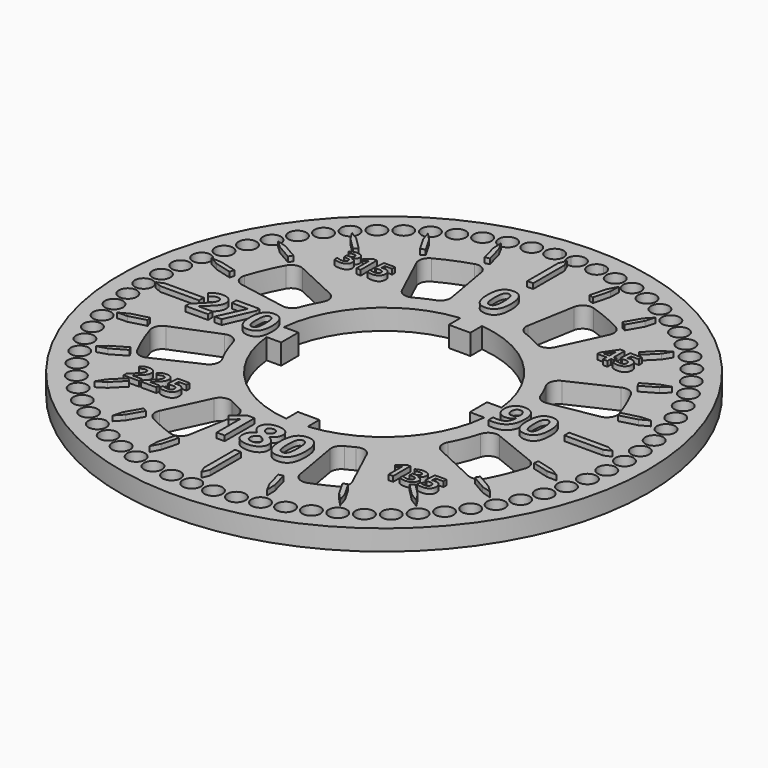
from build123d import *

# Parameters (mm, degrees)
F0_R           = 51.5
F0_R_2         = 1.75
F1_DEPTH       = 4
F3_TEXT_SIZE   = 9.3811322909
F3_TEXT_SIZE_2 = 9.1976195108
F3_TEXT_SIZE_3 = 10.2249465676
F3_TEXT_SIZE_4 = 8.8090639717
F4_DEPTH       = 1
F5_TEXT_SIZE   = 5.8529381123
F5_TEXT_SIZE_2 = 5.8596281128
F5_TEXT_SIZE_3 = 5.9887766838
F5_TEXT_SIZE_4 = 5.5610072903
F6_DEPTH       = 1
F8_DEPTH       = 4.001
F9_R           = 2


# Not quite as in the source:
# - Text() gives the source's letters only with a copy of the font that has no kerning and outlines rounded to 1/6400 em; it was checked with that copy


with BuildPart() as f1:
    # F0 (on Top) → F1 (new body)
    with BuildSketch(Plane.XY):
        Circle(F0_R)
        with Locations((-33.1633080376, -33.1633080376)):
            Circle(F0_R_2, mode=Mode.SUBTRACT)
        with Locations((-30.1467388943, -35.9274843823)):
            Circle(F0_R_2, mode=Mode.SUBTRACT)
        with Locations((-26.9007348649, -38.4182308772)):
            Circle(F0_R_2, mode=Mode.SUBTRACT)
        with Locations((-35.9274843823, -30.1467388943)):
            Circle(F0_R_2, mode=Mode.SUBTRACT)
        with Locations((-38.4182308772, -26.9007348649)):
            Circle(F0_R_2, mode=Mode.SUBTRACT)
        with Locations((-19.8207964756, -42.505835212)):
            Circle(F0_R_2, mode=Mode.SUBTRACT)
        with Locations((-23.45, -40.6165914375)):
            Circle(F0_R_2, mode=Mode.SUBTRACT)
        with Locations((-16.040744722, -44.0715839149)):
            Circle(F0_R_2, mode=Mode.SUBTRACT)
        with Locations((-12.1386132153, -45.301921253)):
            Circle(F0_R_2, mode=Mode.SUBTRACT)
        with Locations((-8.1440995326, -46.1874836163)):
            Circle(F0_R_2, mode=Mode.SUBTRACT)
        with Locations((-4.0876043349, -46.7215313405)):
            Circle(F0_R_2, mode=Mode.SUBTRACT)
        with Locations((0, -46.9)):
            Circle(F0_R_2, mode=Mode.SUBTRACT)
        with Locations((-40.6165914375, -23.45)):
            Circle(F0_R_2, mode=Mode.SUBTRACT)
        with Locations((-42.505835212, -19.8207964756)):
            Circle(F0_R_2, mode=Mode.SUBTRACT)
        with Locations((-44.0715839149, -16.040744722)):
            Circle(F0_R_2, mode=Mode.SUBTRACT)
        with Locations((-45.301921253, -12.1386132153)):
            Circle(F0_R_2, mode=Mode.SUBTRACT)
        with Locations((-46.1874836163, -8.1440995326)):
            Circle(F0_R_2, mode=Mode.SUBTRACT)
        with Locations((-46.7215313405, -4.0876043349)):
            Circle(F0_R_2, mode=Mode.SUBTRACT)
        with Locations((-46.9, 0)):
            Circle(F0_R_2, mode=Mode.SUBTRACT)
        with Locations((4.0876043349, -46.7215313405)):
            Circle(F0_R_2, mode=Mode.SUBTRACT)
        with Locations((8.1440995326, -46.1874836163)):
            Circle(F0_R_2, mode=Mode.SUBTRACT)
        with Locations((12.1386132153, -45.301921253)):
            Circle(F0_R_2, mode=Mode.SUBTRACT)
        with Locations((16.040744722, -44.0715839149)):
            Circle(F0_R_2, mode=Mode.SUBTRACT)
        with Locations((19.8207964756, -42.505835212)):
            Circle(F0_R_2, mode=Mode.SUBTRACT)
        with Locations((23.45, -40.6165914375)):
            Circle(F0_R_2, mode=Mode.SUBTRACT)
        with Locations((26.9007348649, -38.4182308772)):
            Circle(F0_R_2, mode=Mode.SUBTRACT)
        with Locations((30.1467388943, -35.9274843823)):
            Circle(F0_R_2, mode=Mode.SUBTRACT)
        with Locations((33.1633080376, -33.1633080376)):
            Circle(F0_R_2, mode=Mode.SUBTRACT)
        with Locations((35.9274843823, -30.1467388943)):
            Circle(F0_R_2, mode=Mode.SUBTRACT)
        with Locations((38.4182308772, -26.9007348649)):
            Circle(F0_R_2, mode=Mode.SUBTRACT)
        with Locations((40.6165914375, -23.45)):
            Circle(F0_R_2, mode=Mode.SUBTRACT)
        with Locations((42.505835212, -19.8207964756)):
            Circle(F0_R_2, mode=Mode.SUBTRACT)
        with Locations((44.0715839149, -16.040744722)):
            Circle(F0_R_2, mode=Mode.SUBTRACT)
        with Locations((45.301921253, -12.1386132153)):
            Circle(F0_R_2, mode=Mode.SUBTRACT)
        with Locations((46.1874836163, -8.1440995326)):
            Circle(F0_R_2, mode=Mode.SUBTRACT)
        with Locations((46.7215313405, -4.0876043349)):
            Circle(F0_R_2, mode=Mode.SUBTRACT)
        with Locations((46.9, 0)):
            Circle(F0_R_2, mode=Mode.SUBTRACT)
        with Locations((-46.7215313405, 4.0876043349)):
            Circle(F0_R_2, mode=Mode.SUBTRACT)
        with Locations((-46.1874836163, 8.1440995326)):
            Circle(F0_R_2, mode=Mode.SUBTRACT)
        with Locations((-45.301921253, 12.1386132153)):
            Circle(F0_R_2, mode=Mode.SUBTRACT)
        with Locations((-44.0715839149, 16.040744722)):
            Circle(F0_R_2, mode=Mode.SUBTRACT)
        with Locations((-42.505835212, 19.8207964756)):
            Circle(F0_R_2, mode=Mode.SUBTRACT)
        with Locations((-40.6165914375, 23.45)):
            Circle(F0_R_2, mode=Mode.SUBTRACT)
        with BuildLine():
            Line((1.6706053866, 42.8881468691), (1.6706053866, 42.2931905308))
            ThreePointArc((1.6706053866, 42.2931905308), (30.5140559381, 29.3325293461), (42.3261726079, 0))
            ThreePointArc((42.3261726079, 0), (-29.3552011859, -30.4922457514), (-1.6077337049, 42.2956271967))
            Line((-1.6077337049, 42.2956271967), (-1.6077337049, 42.8625403735))
            ThreePointArc((-1.6077337049, 42.8625403735), (-2.9504268896, 43.7092525844), (-3.8994754635, 44.9816728613))
            ThreePointArc((-3.8994754635, 44.9816728613), (-5.8359387226, 46.6451974126), (-4.0518300087, 48.4711656445))
            ThreePointArc((-4.0518300087, 48.4711656445), (0, 51.2457896753), (4.0518300087, 48.4711656445))
            ThreePointArc((4.0518300087, 48.4711656445), (5.3123277586, 47.9715523545), (5.8376043349, 46.7215313405))
            ThreePointArc((5.8376043349, 46.7215313405), (5.2566369424, 45.4192783841), (3.8994754635, 44.9816728613))
            ThreePointArc((3.8994754635, 44.9816728613), (2.9752584659, 43.7323944434), (1.6706053866, 42.8881468691))
        make_face(mode=Mode.SUBTRACT)
        with Locations((-38.4182308772, 26.9007348649)):
            Circle(F0_R_2, mode=Mode.SUBTRACT)
        with Locations((-35.9274843823, 30.1467388943)):
            Circle(F0_R_2, mode=Mode.SUBTRACT)
        with Locations((-33.1633080376, 33.1633080376)):
            Circle(F0_R_2, mode=Mode.SUBTRACT)
        with Locations((-30.1467388943, 35.9274843823)):
            Circle(F0_R_2, mode=Mode.SUBTRACT)
        with Locations((-26.9007348649, 38.4182308772)):
            Circle(F0_R_2, mode=Mode.SUBTRACT)
        with Locations((-23.45, 40.6165914375)):
            Circle(F0_R_2, mode=Mode.SUBTRACT)
        with Locations((-19.8207964756, 42.505835212)):
            Circle(F0_R_2, mode=Mode.SUBTRACT)
        with Locations((-16.040744722, 44.0715839149)):
            Circle(F0_R_2, mode=Mode.SUBTRACT)
        with Locations((-12.1386132153, 45.301921253)):
            Circle(F0_R_2, mode=Mode.SUBTRACT)
        with Locations((-8.1440995326, 46.1874836163)):
            Circle(F0_R_2, mode=Mode.SUBTRACT)
        with Locations((46.7215313405, 4.0876043349)):
            Circle(F0_R_2, mode=Mode.SUBTRACT)
        with Locations((46.1874836163, 8.1440995326)):
            Circle(F0_R_2, mode=Mode.SUBTRACT)
        with Locations((45.301921253, 12.1386132153)):
            Circle(F0_R_2, mode=Mode.SUBTRACT)
        with Locations((44.0715839149, 16.040744722)):
            Circle(F0_R_2, mode=Mode.SUBTRACT)
        with Locations((42.505835212, 19.8207964756)):
            Circle(F0_R_2, mode=Mode.SUBTRACT)
        with Locations((40.6165914375, 23.45)):
            Circle(F0_R_2, mode=Mode.SUBTRACT)
        with Locations((8.1440995326, 46.1874836163)):
            Circle(F0_R_2, mode=Mode.SUBTRACT)
        with Locations((12.1386132153, 45.301921253)):
            Circle(F0_R_2, mode=Mode.SUBTRACT)
        with Locations((16.040744722, 44.0715839149)):
            Circle(F0_R_2, mode=Mode.SUBTRACT)
        with Locations((23.45, 40.6165914375)):
            Circle(F0_R_2, mode=Mode.SUBTRACT)
        with Locations((19.8207964756, 42.505835212)):
            Circle(F0_R_2, mode=Mode.SUBTRACT)
        with Locations((38.4182308772, 26.9007348649)):
            Circle(F0_R_2, mode=Mode.SUBTRACT)
        with Locations((35.9274843823, 30.1467388943)):
            Circle(F0_R_2, mode=Mode.SUBTRACT)
        with Locations((26.9007348649, 38.4182308772)):
            Circle(F0_R_2, mode=Mode.SUBTRACT)
        with Locations((30.1467388943, 35.9274843823)):
            Circle(F0_R_2, mode=Mode.SUBTRACT)
        with Locations((33.1633080376, 33.1633080376)):
            Circle(F0_R_2, mode=Mode.SUBTRACT)
        with BuildLine():
            Line((1.6706053866, 46.3788688819), (1.6706053866, 42.8881468691))
            ThreePointArc((1.6706053866, 42.8881468691), (2.9752584659, 43.7323944434), (3.8994754635, 44.9816728613))
            ThreePointArc((3.8994754635, 44.9816728613), (2.3392699471, 46.7978652684), (4.0518300087, 48.4711656445))
            ThreePointArc((4.0518300087, 48.4711656445), (0, 51.2457896753), (-4.0518300087, 48.4711656445))
            ThreePointArc((-4.0518300087, 48.4711656445), (-2.8375833209, 47.9462547642), (-2.3376043349, 46.7215313405))
            ThreePointArc((-2.3376043349, 46.7215313405), (-2.7853513785, 45.5524987329), (-3.8994754635, 44.9816728613))
            ThreePointArc((-3.8994754635, 44.9816728613), (-2.9504268896, 43.7092525844), (-1.6077337049, 42.8625403735))
            Line((-1.6077337049, 42.8625403735), (-1.6077337049, 46.2088470978))
            ThreePointArc((-1.6077337049, 46.2088470978), (-1.75, 46.9), (-1.6077337049, 47.5911529022))
            Line((-1.6077337049, 47.5911529022), (-1.6077337049, 48.9033423511))
            Line((-1.6077337049, 48.9033423511), (1.6706053866, 48.9033423511))
            Line((1.6706053866, 48.9033423511), (1.6706053866, 47.4211311181))
            ThreePointArc((1.6706053866, 47.4211311181), (1.730037489, 47.1635721661), (1.75, 46.9))
            ThreePointArc((1.75, 46.9), (1.730037489, 46.6364278339), (1.6706053866, 46.3788688819))
        make_face()
        with BuildLine():
            ThreePointArc((-1.6077337049, 42.8625403735), (0.0339431178, 42.5543428844), (1.6706053866, 42.8881468691))
            Line((1.6706053866, 42.8881468691), (1.6706053866, 46.3788688819))
            ThreePointArc((1.6706053866, 46.3788688819), (0.0906369895, 45.1523487373), (-1.6077337049, 46.2088470978))
            Line((-1.6077337049, 46.2088470978), (-1.6077337049, 42.8625403735))
        make_face()
        with BuildLine():
            ThreePointArc((-1.6077337049, 47.5911529022), (0.0906369895, 48.6476512627), (1.6706053866, 47.4211311181))
            Line((1.6706053866, 47.4211311181), (1.6706053866, 48.9033423511))
            Line((1.6706053866, 48.9033423511), (-1.6077337049, 48.9033423511))
            Line((-1.6077337049, 48.9033423511), (-1.6077337049, 47.5911529022))
        make_face()
        with BuildLine():
            ThreePointArc((-1.6077337049, 24.5811957581), (0.0315056688, 24.633696433), (1.6706053866, 24.5770028727))
            Line((1.6706053866, 24.5770028727), (1.6706053866, 27.6260756154))
            ThreePointArc((1.6706053866, 27.6260756154), (0.0314911204, 27.6765240696), (-1.6077337049, 27.629805801))
            Line((-1.6077337049, 27.629805801), (-1.6077337049, 24.5811957581))
        make_face()
        with BuildLine():
            ThreePointArc((-1.6077337049, 24.5811957581), (-16.840658184, -17.9781040294), (24.6337165804, 0))
            ThreePointArc((24.6337165804, 0), (17.999627943, 16.8176510392), (1.6706053866, 24.5770028727))
            ThreePointArc((1.6706053866, 24.5770028727), (0.0315056688, 24.633696433), (-1.6077337049, 24.5811957581))
        make_face()
        with BuildLine():
            ThreePointArc((21.2464702951, 2.1), (21.3241018662, 1.0512752256), (21.35, 0))
            ThreePointArc((21.35, 0), (21.3241018662, -1.0512752256), (21.2464702951, -2.1))
            ThreePointArc((21.2464702951, -2.1), (15.0967297783, -15.0967297783), (2.1, -21.2464702951))
            ThreePointArc((2.1, -21.2464702951), (0, -21.35), (-2.1, -21.2464702951))
            ThreePointArc((-2.1, -21.2464702951), (-15.0967297783, -15.0967297783), (-21.2464702951, -2.1))
            ThreePointArc((-21.2464702951, -2.1), (-21.35, 0), (-21.2464702951, 2.1))
            ThreePointArc((-21.2464702951, 2.1), (-15.0967297783, 15.0967297783), (-2.1, 21.2464702951))
            ThreePointArc((-2.1, 21.2464702951), (0, 21.35), (2.1, 21.2464702951))
            ThreePointArc((2.1, 21.2464702951), (15.0967297783, 15.0967297783), (21.2464702951, 2.1))
        make_face(mode=Mode.SUBTRACT)
        with BuildLine():
            Line((-18.4065936816, 2.1), (-21.2464702951, 2.1))
            ThreePointArc((-21.2464702951, 2.1), (-21.35, 0), (-21.2464702951, -2.1))
            Line((-21.2464702951, -2.1), (-18.4065936816, -2.1))
            Line((-18.4065936816, -2.1), (-18.4065936816, 2.1))
        make_face()
        with BuildLine():
            Line((2.1, 18.4065936816), (2.1, 21.2464702951))
            ThreePointArc((2.1, 21.2464702951), (0, 21.35), (-2.1, 21.2464702951))
            Line((-2.1, 21.2464702951), (-2.1, 18.4065936816))
            Line((-2.1, 18.4065936816), (2.1, 18.4065936816))
        make_face()
        with BuildLine():
            ThreePointArc((21.2464702951, -2.1), (21.3241018662, -1.0512752256), (21.35, 0))
            ThreePointArc((21.35, 0), (21.3241018662, 1.0512752256), (21.2464702951, 2.1))
            Line((21.2464702951, 2.1), (18.4065936816, 2.1))
            Line((18.4065936816, 2.1), (18.4065936816, -2.1))
            Line((18.4065936816, -2.1), (21.2464702951, -2.1))
        make_face()
        with BuildLine():
            ThreePointArc((-2.1, -21.2464702951), (0, -21.35), (2.1, -21.2464702951))
            Line((2.1, -21.2464702951), (2.1, -18.4065936816))
            Line((2.1, -18.4065936816), (-2.1, -18.4065936816))
            Line((-2.1, -18.4065936816), (-2.1, -21.2464702951))
        make_face()
        with BuildLine():
            Line((1.6706053866, 42.2931905308), (1.6706053866, 27.6260756154))
            ThreePointArc((1.6706053866, 27.6260756154), (20.1522648403, 18.97042957), (27.6765419853, 0))
            ThreePointArc((27.6765419853, 0), (-18.9933470837, -20.1306667258), (-1.6077337049, 27.629805801))
            Line((-1.6077337049, 27.629805801), (-1.6077337049, 42.2956271967))
            ThreePointArc((-1.6077337049, 42.2956271967), (-29.3552011859, -30.4922457514), (42.3261726079, 0))
            ThreePointArc((42.3261726079, 0), (30.5140559381, 29.3325293461), (1.6706053866, 42.2931905308))
        make_face()
        with BuildLine():
            ThreePointArc((1.6706053866, 24.5770028727), (17.999627943, 16.8176510392), (24.6337165804, 0))
            ThreePointArc((24.6337165804, 0), (-16.840658184, -17.9781040294), (-1.6077337049, 24.5811957581))
            Line((-1.6077337049, 24.5811957581), (-1.6077337049, 27.629805801))
            ThreePointArc((-1.6077337049, 27.629805801), (-18.9933470837, -20.1306667258), (27.6765419853, 0))
            ThreePointArc((27.6765419853, 0), (20.1522648403, 18.97042957), (1.6706053866, 27.6260756154))
            Line((1.6706053866, 27.6260756154), (1.6706053866, 24.5770028727))
        make_face()
        with BuildLine():
            ThreePointArc((-1.6077337049, 27.629805801), (0.0314911204, 27.6765240696), (1.6706053866, 27.6260756154))
            Line((1.6706053866, 27.6260756154), (1.6706053866, 42.2931905308))
            ThreePointArc((1.6706053866, 42.2931905308), (0.031459441, 42.3261609166), (-1.6077337049, 42.2956271967))
            Line((-1.6077337049, 42.2956271967), (-1.6077337049, 27.629805801))
        make_face()
        with BuildLine():
            ThreePointArc((-1.6077337049, 42.2956271967), (0.031459441, 42.3261609166), (1.6706053866, 42.2931905308))
            Line((1.6706053866, 42.2931905308), (1.6706053866, 42.8881468691))
            ThreePointArc((1.6706053866, 42.8881468691), (0.0339431178, 42.5543428844), (-1.6077337049, 42.8625403735))
            Line((-1.6077337049, 42.8625403735), (-1.6077337049, 42.2956271967))
        make_face()
    extrude(amount=F1_DEPTH)

    # F3 (on face) → F4 (join)
    with BuildSketch(Plane.XY.offset(4)):
        Polygon((0.5807150155, 43.2173013687), (0, 43.2173013687), (-0.5807150155, 43.2173013687), (-0.5807150155, 35.6378108263), (0, 35.6378108263), (0.5807150155, 35.6378108263), align=None)
        Polygon((-0.5807150155, 43.2173013687), (0, 43.2173013687), (0.5807150155, 43.2173013687), (0, 44.5837080479), align=None)
        Polygon((-44.5837080479, 0), (-43.2173013687, -0.5807150155), (-35.6378108263, -0.5807150155), (-35.6378108263, 0), (-35.6378108263, 0.5807150155), (-43.2173013687, 0.5807150155), align=None)
        Polygon((0, -44.5837080479), (0.5807150155, -43.2173013687), (0.5807150155, -35.6378108263), (0, -35.6378108263), (-0.5807150155, -35.6378108263), (-0.5807150155, -43.2173013687), align=None)
        Polygon((44.5837080479, 0), (43.2173013687, 0.5807150155), (35.6378108263, 0.5807150155), (35.6378108263, 0), (35.6378108263, -0.5807150155), (43.2173013687, -0.5807150155), align=None)
        with Locations((-2.8143396873, 24.9150719494)):
            Text('0', F3_TEXT_SIZE, font='Open Sans', font_style=FontStyle.BOLD, text_align=(TextAlign.LEFT, TextAlign.BOTTOM))
        with Locations((22.7051582187, -3.8054117467)):
            Text('90', F3_TEXT_SIZE_2, font='Open Sans', font_style=FontStyle.BOLD, text_align=(TextAlign.LEFT, TextAlign.BOTTOM))
        with Locations((-8.9881005879, -32.929463312)):
            Text('180', F3_TEXT_SIZE_3, font='Open Sans', font_style=FontStyle.BOLD, text_align=(TextAlign.LEFT, TextAlign.BOTTOM))
        with Locations((-36.4714260625, -3.2847125136)):
            Text('270', F3_TEXT_SIZE_4, font='Open Sans', font_style=FontStyle.BOLD, text_align=(TextAlign.LEFT, TextAlign.BOTTOM))
    extrude(amount=F4_DEPTH)

    # F5 (on face) → F6 (join)
    with BuildSketch(Plane.XY.offset(4)):
        Polygon((29.7286761925, 30.3481696174), (27.3688435555, 27.9883369803), (28.0026486143, 27.3545319214), (30.3624812514, 29.7143645585), align=None)
        Polygon((31.3885398209, 31.3885398209), (29.7286761925, 30.3481696174), (30.3624812514, 29.7143645585), align=None)
        Polygon((20.8610118347, 37.0084283983), (19.1923581746, 34.1182354788), (19.96860767, 33.6700676237), (21.6372613301, 36.5602605432), (22.1950493589, 38.4429531661), align=None)
        Polygon((10.5717039949, 41.1466239432), (9.7079453011, 37.9230326124), (10.5737391126, 37.6910438598), (11.4374978064, 40.9146351906), (11.4890029622, 42.8775427831), align=None)
        Polygon((-0.4380480016, 42.4807450644), (-0.4380480016, 39.1434377442), (0.4582877086, 39.1434377442), (0.4582877086, 42.4807450644), (0, 44.3900987178), align=None)
        Polygon((-11.4179477508, 40.9198736122), (-10.5541890569, 37.6962822814), (-9.6883952454, 37.928271034), (-10.5521539393, 41.1518623648), (-11.4890029622, 42.8775427831), align=None)
        Polygon((-21.6197332297, 36.5703803967), (-19.9510795696, 33.6801874771), (-19.1748300743, 34.1283553322), (-20.8434837344, 37.0185482518), (-22.1950493589, 38.4429531661), align=None)
        Polygon((-30.3481696174, 29.7286761925), (-27.9883369803, 27.3688435555), (-27.3545319214, 28.0026486143), (-29.7143645585, 30.3624812514), (-31.3885398209, 31.3885398209), align=None)
        Polygon((-37.0084283983, 20.8610118347), (-34.1182354788, 19.1923581746), (-33.6700676237, 19.96860767), (-36.5602605432, 21.6372613301), (-38.4429531661, 22.1950493589), align=None)
        Polygon((-41.1466239432, 10.5717039949), (-37.9230326124, 9.7079453011), (-37.6910438598, 10.5737391126), (-40.9146351906, 11.4374978064), (-42.8775427831, 11.4890029622), align=None)
        Polygon((-42.4807450644, -0.4380480016), (-39.1434377442, -0.4380480016), (-39.1434377442, 0.4582877086), (-42.4807450644, 0.4582877086), (-44.3900987178, 0), align=None)
        Polygon((-40.9198736122, -11.4179477508), (-37.6962822814, -10.5541890569), (-37.928271034, -9.6883952454), (-41.1518623648, -10.5521539393), (-42.8775427831, -11.4890029622), align=None)
        Polygon((-36.5703803967, -21.6197332297), (-33.6801874771, -19.9510795696), (-34.1283553322, -19.1748300743), (-37.0185482518, -20.8434837344), (-38.4429531661, -22.1950493589), align=None)
        Polygon((-29.7286761925, -30.3481696174), (-27.3688435555, -27.9883369803), (-28.0026486143, -27.3545319214), (-30.3624812514, -29.7143645585), (-31.3885398209, -31.3885398209), align=None)
        Polygon((-20.8610118347, -37.0084283983), (-19.1923581746, -34.1182354788), (-19.96860767, -33.6700676237), (-21.6372613301, -36.5602605432), (-22.1950493589, -38.4429531661), align=None)
        Polygon((-10.5717039949, -41.1466239432), (-9.7079453011, -37.9230326124), (-10.5737391126, -37.6910438598), (-11.4374978064, -40.9146351906), (-11.4890029622, -42.8775427831), align=None)
        Polygon((0.4380480016, -42.4807450644), (0.4380480016, -39.1434377442), (-0.4582877086, -39.1434377442), (-0.4582877086, -42.4807450644), (0, -44.3900987178), align=None)
        Polygon((11.4179477508, -40.9198736122), (10.5541890569, -37.6962822814), (9.6883952454, -37.928271034), (10.5521539393, -41.1518623648), (11.4890029622, -42.8775427831), align=None)
        Polygon((21.6197332297, -36.5703803967), (19.9510795696, -33.6801874771), (19.1748300743, -34.1283553322), (20.8434837344, -37.0185482518), (22.1950493589, -38.4429531661), align=None)
        Polygon((30.3481696174, -29.7286761925), (27.9883369803, -27.3688435555), (27.3545319214, -28.0026486143), (29.7143645585, -30.3624812514), (31.3885398209, -31.3885398209), align=None)
        Polygon((37.0084283983, -20.8610118347), (34.1182354788, -19.1923581746), (33.6700676237, -19.96860767), (36.5602605432, -21.6372613301), (38.4429531661, -22.1950493589), align=None)
        Polygon((41.1466239432, -10.5717039949), (37.9230326124, -9.7079453011), (37.6910438598, -10.5737391126), (40.9146351906, -11.4374978064), (42.8775427831, -11.4890029622), align=None)
        Polygon((42.4807450644, 0.4380480016), (39.1434377442, 0.4380480016), (39.1434377442, -0.4582877086), (42.4807450644, -0.4582877086), (44.3900987178, 0), align=None)
        Polygon((40.9198736122, 11.4179477508), (37.6962822814, 10.5541890569), (37.928271034, 9.6883952454), (41.1518623648, 10.5521539393), (42.8775427831, 11.4890029622), align=None)
        Polygon((36.5703803967, 21.6197332297), (33.6801874771, 19.9510795696), (34.1283553322, 19.1748300743), (37.0185482518, 20.8434837344), (38.4429531661, 22.1950493589), align=None)
        with Locations((22.6847687736, 22.6847687736)):
            Text('45', F5_TEXT_SIZE, font='Open Sans', font_style=FontStyle.BOLD, text_align=(TextAlign.LEFT, TextAlign.BOTTOM))
        with Locations((21.2376496824, -27.3688435555)):
            Text('135', F5_TEXT_SIZE_2, font='Open Sans', font_style=FontStyle.BOLD, text_align=(TextAlign.LEFT, TextAlign.BOTTOM))
        with Locations((-29.4221136719, -27.028683573)):
            Text('225', F5_TEXT_SIZE_3, font='Open Sans', font_style=FontStyle.BOLD, text_align=(TextAlign.LEFT, TextAlign.BOTTOM))
        with Locations((-28.1775593758, 22.6847687736)):
            Text('315', F5_TEXT_SIZE_4, font='Open Sans', font_style=FontStyle.BOLD, text_align=(TextAlign.LEFT, TextAlign.BOTTOM))
    extrude(amount=F6_DEPTH)

    # F7 (on face) → F8 (cut, through all)
    with BuildSketch(Plane.XY.offset(4)):
        with BuildLine():
            ThreePointArc((-13.8661036658, 20.8713257789), (-10.6000719036, 22.7050555224), (-7.0971895416, 24.031457951))
            Line((-7.0971895416, 24.031457951), (-9.4090410933, 37.1426196256))
            ThreePointArc((-9.4090410933, 37.1426196256), (-14.6091752326, 35.4214094294), (-19.5107385419, 32.9762843343))
            Line((-19.5107385419, 32.9762843343), (-13.8661036658, 20.8713257789))
        make_face()
        with BuildLine():
            ThreePointArc((7.1855451351, 24.0051871842), (10.8151856558, 22.6033809389), (14.1840524408, 20.6565661957))
            Line((14.1840524408, 20.6565661957), (19.8376201997, 32.7806813803))
            ThreePointArc((19.8376201997, 32.7806813803), (14.8274235478, 35.3306065314), (9.4980338318, 37.1199622882))
            Line((9.4980338318, 37.1199622882), (7.1855451351, 24.0051871842))
        make_face()
        with BuildLine():
            Line((23.9809782551, 7.2659309498), (37.0991463846, 9.5790179285))
            ThreePointArc((37.0991463846, 9.5790179285), (35.4023857825, 14.6552150394), (33.0148267345, 19.4454483784))
            Line((33.0148267345, 19.4454483784), (20.9134522402, 13.8024847776))
            ThreePointArc((20.9134522402, 13.8024847776), (22.6838953084, 10.6452789667), (23.9809782551, 7.2659309498))
        make_face()
        with BuildLine():
            ThreePointArc((33.0249817089, -19.4281967787), (35.4166692631, -14.6206629554), (37.1127979572, -9.5259894357))
            Line((37.1127979572, -9.5259894357), (24.6517429206, -4.4913963993))
            ThreePointArc((24.6517429206, -4.4913963993), (23.2571555863, -9.3266170006), (20.9245409192, -13.7856685714))
            Line((20.9245409192, -13.7856685714), (33.0249817089, -19.4281967787))
        make_face()
        with BuildLine():
            Line((19.5785274741, -32.9360821728), (13.9321178673, -20.827317695))
            ThreePointArc((13.9321178673, -20.827317695), (11.5803656083, -22.2210756494), (9.0907790531, -23.3503491804))
            Line((9.0907790531, -23.3503491804), (11.4224061947, -36.5736637988))
            ThreePointArc((11.4224061947, -36.5736637988), (15.6068085176, -34.9933104298), (19.5785274741, -32.9360821728))
        make_face()
        with BuildLine():
            Line((-10.7044652009, -36.7901980384), (-8.3812038409, -23.6143281254))
            ThreePointArc((-8.3812038409, -23.6143281254), (-11.2367312556, -22.3968064984), (-13.9198030985, -20.8355502049))
            Line((-13.9198030985, -20.8355502049), (-19.5658784877, -32.9435979509))
            ThreePointArc((-19.5658784877, -32.9435979509), (-15.2568840139, -35.1472863409), (-10.7044652009, -36.7901980384))
        make_face()
        with BuildLine():
            Line((-32.9414073416, -19.5695664055), (-20.8331509383, -13.9233937178))
            ThreePointArc((-20.8331509383, -13.9233937178), (-23.2313987179, -9.3905901971), (-24.6566326054, -4.4644752436))
            Line((-24.6566326054, -4.4644752436), (-37.1195092385, -9.4998042527))
            ThreePointArc((-37.1195092385, -9.4998042527), (-35.3904370623, -14.684046155), (-32.9414073416, -19.5695664055))
        make_face()
        with BuildLine():
            ThreePointArc((-24.0273049966, 7.1112365478), (-22.6208642703, 10.7785699565), (-20.6586155087, 14.1810675163))
            Line((-20.6586155087, 14.1810675163), (-32.7825410592, 19.8345468475))
            ThreePointArc((-32.7825410592, 19.8345468475), (-35.3462265275, 14.7901493303), (-37.1390330447, 9.4231879664))
            Line((-37.1390330447, 9.4231879664), (-24.0273049966, 7.1112365478))
        make_face()
    extrude(amount=-F8_DEPTH, mode=Mode.SUBTRACT)

    # F9
    f9_edges = [f1.edges().sort_by_distance(p)[0] for p in [
        (-13.866104, 20.871326, 2),
        (-7.09719, 24.031458, 2),
        (-19.510739, 32.976284, 2),
        (-9.409041, 37.14262, 2),
        (9.498034, 37.119962, 2),
        (19.83762, 32.780681, 2),
        (7.185545, 24.005187, 2),
        (14.184052, 20.656566, 2),
        (20.913452, 13.802485, 2),
        (37.099146, 9.579018, 2),
        (33.014827, 19.445448, 2),
        (23.980978, 7.265931, 2),
        (24.651743, -4.491396, 2),
        (37.112798, -9.525989, 2),
        (20.924541, -13.785669, 2),
        (33.024982, -19.428197, 2),
        (13.932118, -20.827318, 2),
        (9.090779, -23.350349, 2),
        (19.578527, -32.936082, 2),
        (11.422406, -36.573664, 2),
        (-19.565878, -32.943598, 2),
        (-13.919803, -20.83555, 2),
        (-8.381204, -23.614328, 2),
        (-10.704465, -36.790198, 2),
        (-24.656633, -4.464475, 2),
        (-32.941407, -19.569566, 2),
        (-20.833151, -13.923394, 2),
        (-37.119509, -9.499804, 2),
        (-24.027305, 7.111237, 2),
        (-37.139033, 9.423188, 2),
        (-32.782541, 19.834547, 2),
        (-20.658616, 14.181068, 2),
    ]]
    fillet(f9_edges, radius=F9_R)


solid = f1.part
